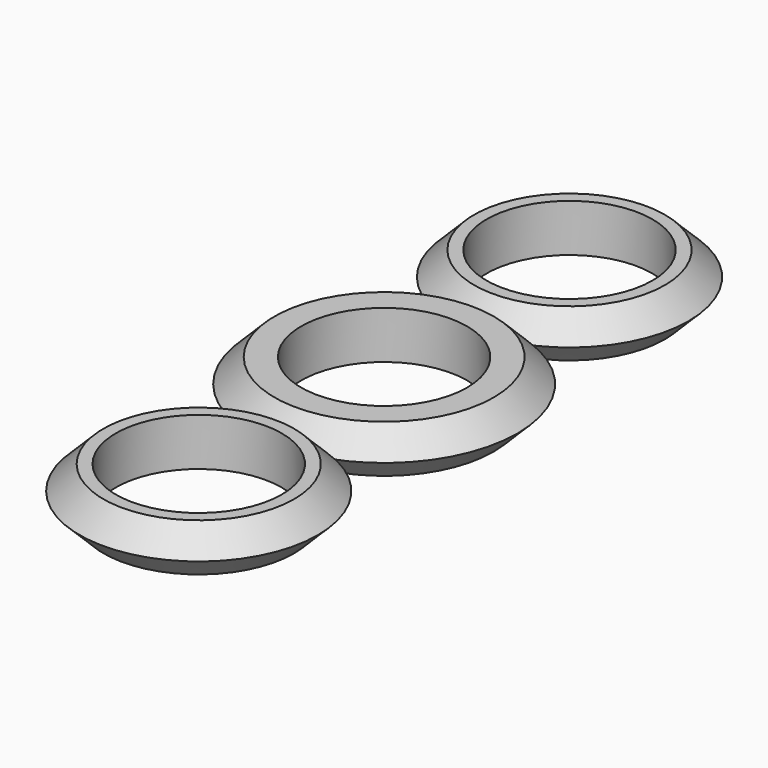
from build123d import *

# Parameters (mm, degrees)
F1_R      = 17.78
F1_R_2    = 11.049
F3_DEPTH  = 6.35
F2_R      = 19.685
F2_R_2    = 11.049
F0_R      = 17.78
F0_R_2    = 11.049
F4_SIZE   = 5.08
F4_2_SIZE = 5.08
F4_3_SIZE = 5.08


# Not quite as in the source:
# - a fillet or chamfer that OpenCascade refuses, or shapes differently, is made with other operations: its cross-section is extruded or revolved along the edge and cut away or added


with BuildPart() as f3:
    # F1 (on Top) → F3 (new body)
    with BuildSketch(Plane.XY):
        with Locations((0, 30.8565702289)):
            Circle(F1_R)
        with Locations((0, 30.8565702289)):
            Circle(F1_R_2, mode=Mode.SUBTRACT)
    extrude(amount=F3_DEPTH)

    # F4
    f4_edges = [f3.edges().sort_by_distance(p)[0] for p in [
        (-17.78, 30.85657, 0),
    ]]
    chamfer(f4_edges, length=F4_SIZE)

    # F5: chamfer of 5.08 on 1 edges, made by hand

    # F5_s1 → F5_t2 (revolve, cut)
    with BuildSketch(Plane.XZ.offset(-30.8565702289)):
        Polygon((17.78, 1.27), (12.7, 6.35), (17.78, 6.35), align=None)
    revolve(axis=Axis((0, 30.8565702289, 6.35), (0, 0, 1)), mode=Mode.SUBTRACT)


with BuildPart() as f3b:
    # F2 (on Top) → F3, piece 2 (new body)
    with BuildSketch(Plane.XY):
        Circle(F2_R)
        Circle(F2_R_2, mode=Mode.SUBTRACT)
    extrude(amount=F3_DEPTH)

    # F4#2
    f4_2_edges = [f3b.edges().sort_by_distance(p)[0] for p in [
        (-19.685, 0, 0),
    ]]
    chamfer(f4_2_edges, length=F4_2_SIZE)

    # F5#2: chamfer of 5.08 on 1 edges, made by hand

    # F5_2_s1 → F5_2_t2 (revolve, cut)
    with BuildSketch(Plane.XZ):
        Polygon((19.685, 1.27), (14.605, 6.35), (19.685, 6.35), align=None)
    revolve(axis=Axis((0, 0, 6.35), (0, 0, 1)), mode=Mode.SUBTRACT)


with BuildPart() as f3c:
    # F0 (on Top) → F3, piece 3 (new body)
    with BuildSketch(Plane.XY):
        with Locations((0, -30.8565702289)):
            Circle(F0_R)
        with Locations((0, -30.8565702289)):
            Circle(F0_R_2, mode=Mode.SUBTRACT)
    extrude(amount=F3_DEPTH)

    # F4#3
    f4_3_edges = [f3c.edges().sort_by_distance(p)[0] for p in [
        (-17.78, -30.85657, 0),
    ]]
    chamfer(f4_3_edges, length=F4_3_SIZE)

    # F5#3: chamfer of 5.08 on 1 edges, made by hand

    # F5_3_s1 → F5_3_t2 (revolve, cut)
    with BuildSketch(Plane.XZ.offset(30.8565702289)):
        Polygon((17.78, 1.27), (12.7, 6.35), (17.78, 6.35), align=None)
    revolve(axis=Axis((0, -30.8565702289, 6.35), (0, 0, 1)), mode=Mode.SUBTRACT)


solid = Compound([f3.part, f3b.part, f3c.part])
